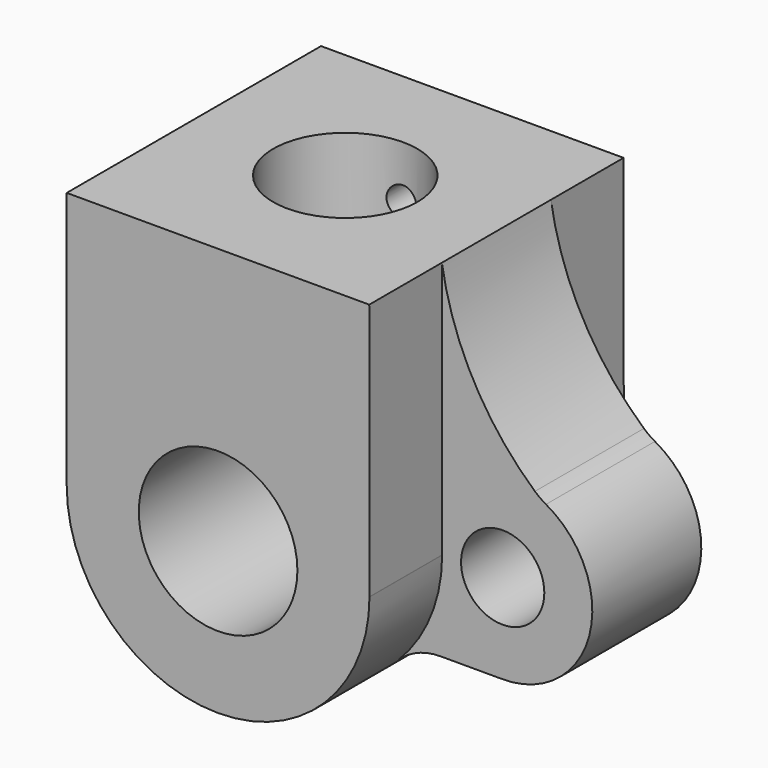
from build123d import *

# Parameters (mm, degrees)
F0_R      = 63.5
F0_R_2    = 16.637
F1_DEPTH  = 66.675
F2_R      = 63.5
F2_R_2    = 8.73125
F3_DEPTH  = 66.676
F4_R      = 8.73125
F5_DEPTH  = 19.05
F7_R      = 15.1150654982
F8_DEPTH  = 53.594
F9_R      = 3.175
F10_DEPTH = 25.4


# Not quite as in the source:
# - a pattern or mirror of a feature is missing from the dataset's text; its kind, count and spacing are read off the source's solid


with BuildPart() as f1:
    # F0 (on Front) → F1 (new body)
    with BuildSketch(Plane.XZ):
        Circle(F0_R)
        Circle(F0_R_2, mode=Mode.SUBTRACT)
    extrude(amount=F1_DEPTH)

    # F2 (on face) → F3 (cut, through all)
    with BuildSketch(Plane.XZ.offset(66.675)):
        Circle(F2_R)
        with BuildLine():
            Line((-31.75, 0), (-31.75, 53.975))
            Line((-31.75, 53.975), (31.7028198831, 53.975))
            ThreePointArc((31.7028198831, 53.975), (38.3398958316, 34.3431316591), (51.2105212065, 18.1009632644))
            ThreePointArc((51.2105212065, 18.1009632644), (52.3246389461, 17.2136710516), (53.5311013852, 16.4567072537))
            ThreePointArc((53.5311013852, 16.4567072537), (62.6217032006, -4.8040419219), (44.2117641598, -18.7944901416))
            Line((44.2117641598, -18.7944901416), (31.3671737764, -18.7944901416))
            ThreePointArc((31.3671737764, -18.7944901416), (26.5189786011, -19.756304441), (22.405124126, -22.4960643869))
            ThreePointArc((22.405124126, -22.4960643869), (-12.179897557, -29.3208559817), (-31.75, 0))
        make_face(mode=Mode.SUBTRACT)
        with Locations((44.45, 0)):
            Circle(F2_R_2)
    extrude(amount=-F3_DEPTH, mode=Mode.SUBTRACT)

    # F4 (on face) → F5 (cut)
    with BuildSketch(Plane.XZ.offset(66.675)):
        with BuildLine():
            Line((31.3671737764, -18.7944901416), (44.2117641598, -18.7944901416))
            ThreePointArc((44.2117641598, -18.7944901416), (62.6217032006, -4.8040419219), (53.5311013852, 16.4567072537))
            ThreePointArc((53.5311013852, 16.4567072537), (52.3246389461, 17.2136710516), (51.2105212065, 18.1009632644))
            ThreePointArc((51.2105212065, 18.1009632644), (38.3398958316, 34.3431316591), (31.7028198831, 53.975))
            Line((31.7028198831, 53.975), (31.7499514816, 0.0555059775))
            ThreePointArc((31.7499514816, 0.0555059775), (31.7499878704, 0.0277529994), (31.75, 0))
            ThreePointArc((31.75, 0), (29.3208559817, -12.179897557), (22.405124126, -22.4960643869))
            ThreePointArc((22.405124126, -22.4960643869), (26.5189786011, -19.756304441), (31.3671737764, -18.7944901416))
        make_face()
        with Locations((44.45, 0)):
            Circle(F4_R, mode=Mode.SUBTRACT)
    f5 = extrude(amount=-F5_DEPTH, mode=Mode.SUBTRACT)

    # F5_copies: F5 across plane
    add(f5.mirror(Plane.ZX.offset(-33.3375)), mode=Mode.SUBTRACT)

    # F7 (on face) → F8 (cut)
    with BuildSketch(Plane.XY.offset(53.975)):
        with Locations((0, -33.3375)):
            Circle(F7_R)
    extrude(amount=-F8_DEPTH, mode=Mode.SUBTRACT)

    # F9 (on face) → F10 (cut)
    with BuildSketch(Plane(origin=(0, 0, 0), x_dir=(-1, 0, 0), z_dir=(0, 1, 0))):
        with Locations((0, 42.8625)):
            Circle(F9_R)
    extrude(amount=-F10_DEPTH, mode=Mode.SUBTRACT)


solid = f1.part
